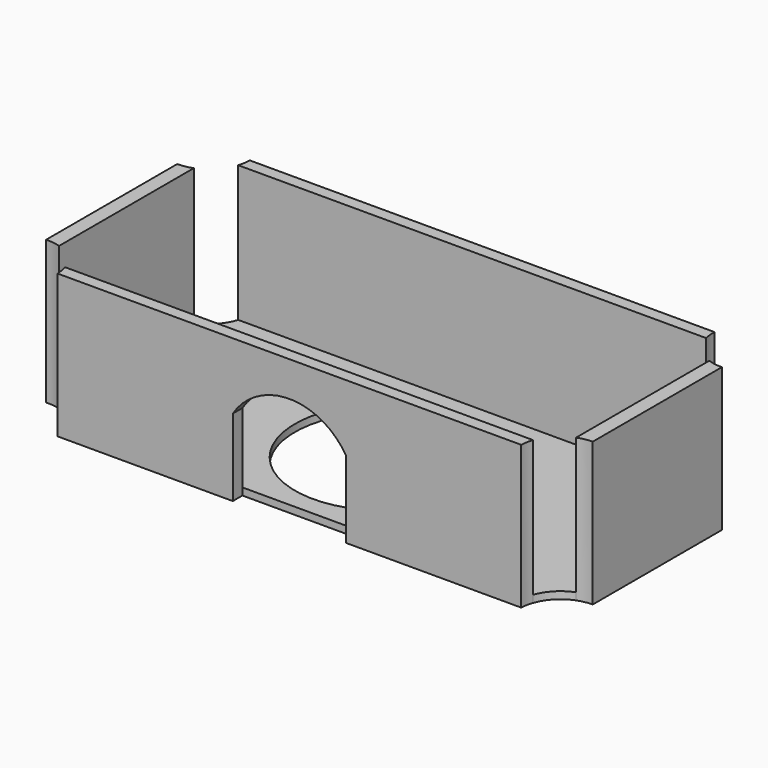
from build123d import *

# Parameters (mm, degrees)
F1_DEPTH = 25.4
F4_DEPTH = 2.286
F0_R     = 16.0333450032
F6_DEPTH = 1.27


# Not quite as in the source:
# - the program builds the solid bodies; features that only make, move or delete a surface that nothing else refers to are left out


with BuildPart() as f1:
    # F0 (on Top) → F1 (new body)
    with BuildSketch(Plane.XY):
        with BuildLine():
            ThreePointArc((41.2870626156, 19.4157604128), (41.1100626555, 20.4737561097), (41.0935558069, 21.5463284403))
            Line((41.0935558069, 21.5463284403), (-41.2941743717, 21.5463284403))
            ThreePointArc((-41.2941743717, 21.5463284403), (-41.3759617074, 20.468700907), (-41.6194500738, 19.4157604128))
            Line((-41.6194500738, 19.4157604128), (41.2870626156, 19.4157604128))
        make_face()
    extrude(amount=F1_DEPTH)


with BuildPart() as f1b:
    # F0 (on Top) → F1, piece 2 (new body)
    with BuildSketch(Plane.XY):
        with BuildLine():
            ThreePointArc((-45.8724014461, 14.8815286098), (-47.1315574375, 14.5259187823), (-48.4344623983, 14.4060404137))
            Line((-48.4344623983, 14.4060404137), (-48.4344623983, -14.6258958917))
            ThreePointArc((-48.4344623983, -14.6258958917), (-47.1390504435, -14.6669589449), (-45.8724014461, -14.9415106237))
            Line((-45.8724014461, -14.9415106237), (-45.8724014461, 14.8815286098))
        make_face()
    extrude(amount=F1_DEPTH)


with BuildPart() as f1c:
    # F0 (on Top) → F1, piece 3 (new body)
    with BuildSketch(Plane.XY):
        with BuildLine():
            ThreePointArc((41.2976550473, -21.5463284403), (41.4141256039, -20.4659523028), (41.6931864989, -19.4157604128))
            Line((41.6931864989, -19.4157604128), (-41.2653559278, -19.4157604128))
            ThreePointArc((-41.2653559278, -19.4157604128), (-40.9888024923, -20.4661473001), (-40.8747712689, -21.5463284403))
            Line((-40.8747712689, -21.5463284403), (41.2976550473, -21.5463284403))
        make_face()
    extrude(amount=F1_DEPTH)

    # F3 (on face) → F4 (cut)
    with BuildSketch(Plane.XZ.offset(21.5463284403)):
        with BuildLine():
            Line((-9.814559482, 13.6550404131), (-9.814559482, 0))
            Line((-9.814559482, 0), (10.2412803099, 0))
            Line((10.2412803099, 0), (10.2412803099, 13.6550404131))
            ThreePointArc((10.2412803099, 13.6550404131), (0.2133604139, 19.2100995282), (-9.814559482, 13.6550404131))
        make_face()
    extrude(amount=-F4_DEPTH, mode=Mode.SUBTRACT)


with BuildPart() as f1d:
    # F0 (on Top) → F1, piece 4 (new body)
    with BuildSketch(Plane.XY):
        with BuildLine():
            Line((48.4344623983, -14.6289617851), (48.4344623983, 13.9825086435))
            ThreePointArc((48.4344623983, 13.9825086435), (47.135395826, 14.0623418721), (45.8724014461, 14.3766546148))
            Line((45.8724014461, 14.3766546148), (45.8724014461, -15.1044499813))
            ThreePointArc((45.8724014461, -15.1044499813), (47.1315574375, -14.7488401538), (48.4344623983, -14.6289617851))
        make_face()
    extrude(amount=F1_DEPTH)


with BuildPart() as f6:
    # F0 (on Top) → F6 (new body)
    with BuildSketch(Plane.XY):
        with BuildLine():
            ThreePointArc((45.8724014461, 14.3766546148), (42.9399574045, 16.31404402), (41.2870626156, 19.4157604128))
            Line((41.2870626156, 19.4157604128), (-41.6194500738, 19.4157604128))
            ThreePointArc((-41.6194500738, 19.4157604128), (-43.2265654792, 16.6615026724), (-45.8724014461, 14.8815286098))
            Line((-45.8724014461, 14.8815286098), (-45.8724014461, -14.9415106237))
            ThreePointArc((-45.8724014461, -14.9415106237), (-43.0374644665, -16.6314489243), (-41.2653559278, -19.4157604128))
            Line((-41.2653559278, -19.4157604128), (41.6931864989, -19.4157604128))
            ThreePointArc((41.6931864989, -19.4157604128), (43.3075853222, -16.7994566018), (45.8724014461, -15.1044499813))
            Line((45.8724014461, -15.1044499813), (45.8724014461, 14.3766546148))
        make_face()
        Circle(F0_R, mode=Mode.SUBTRACT)
    extrude(amount=F6_DEPTH)


solid = Compound([f1.part, f1b.part, f1c.part, f1d.part, f6.part])
